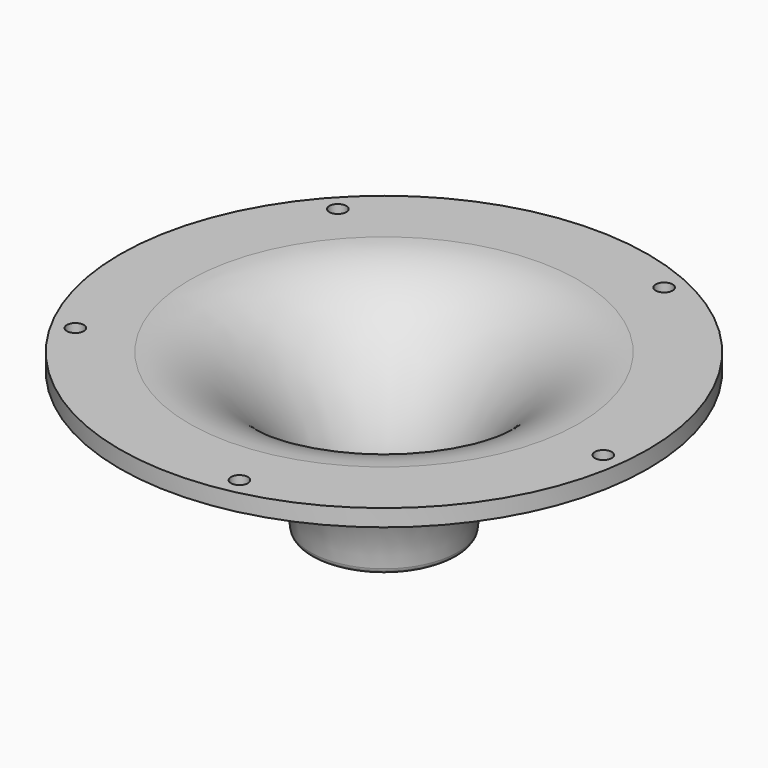
from build123d import *

# Parameters (mm, degrees)
F3_D            = 3
F3_COPIES_COUNT = 5
F5_R            = 1


# Not quite as in the source:
# - a pattern or mirror of a feature is missing from the dataset's text; its kind, count and spacing are read off the source's solid


with BuildPart() as f1:
    # F0 (on Front) → F1 (revolve)
    with BuildSketch(Plane.XZ):
        with BuildLine():
            Line((-34.4849, 28), (-46.8049, 28))
            Line((-46.8049, 28), (-46.8049, 25))
            Line((-46.8049, 25), (-34.4849, 25))
            add(Edge.make_bspline(
                [(-34.4849, 25), (-23.5746630862, 25), (-12.9841, 10.9102369138), (-12.9841, 0)],
                knots=[0, 0, 0, 0, 32.9739958246, 32.9739958246, 32.9739958246, 32.9739958246], degree=3))
            Line((-12.9841, 0), (-10.805, 0))
            add(Edge.make_bspline(
                [(-34.4849, 28), (-22.341688069, 28), (-10.805, 12.143211931), (-10.805, 0)],
                knots=[0, 0, 0, 0, 36.6706648973, 36.6706648973, 36.6706648973, 36.6706648973], degree=3))
        make_face()
    revolve(axis=Axis((0, 0, 25.7415452758), (0, 0, 1)))

    # F3 (through all)
    with Locations(Plane(origin=(0, 0, 0), x_dir=(1, 0, 0), z_dir=(0, 0, -1))):
        with Locations((-31.7452536422, -29.4542566568)):
            f3 = Hole(F3_D / 2)

    # F3_copies: F3 ×5 about axis
    f3_copies_axis = Axis((0, 0, 0), (0, 0, 1))
    for i in range(1, F3_COPIES_COUNT):
        add(f3.rotate(f3_copies_axis, i * 360 / F3_COPIES_COUNT), mode=Mode.SUBTRACT)

    # F5
    f5_edges = [f1.edges().sort_by_distance(p)[0] for p in [
        (12.9841, 0, 0),
        (10.805, 0, 0),
    ]]
    fillet(f5_edges, radius=F5_R)


solid = f1.part
